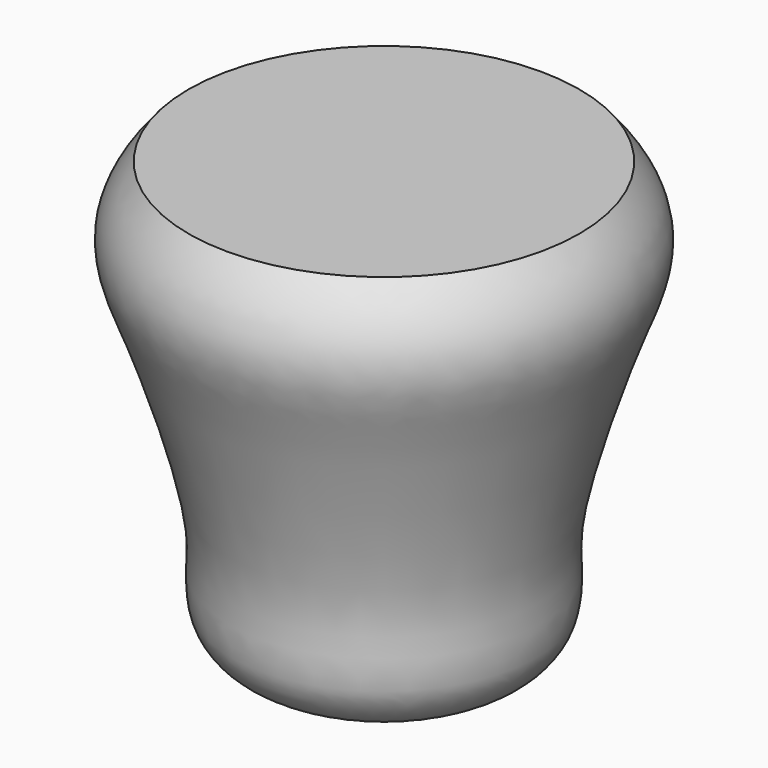
from build123d import *


with BuildPart() as f1:
    # F0 (on Right) → F1 (revolve)
    with BuildSketch(Plane.YZ):
        with BuildLine():
            Line((40, 90), (0, 90))
            Line((0, 90), (0, 0))
            Line((0, 0), (20, 0))
            add(Edge.make_bspline(
                [(40, 90), (49.5818336765, 78.8694407024), (42.4350350409, 64.2002089946), (33.3484499065, 35.488516994), (30.97101949, 21.463351906), (32.5174405975, 10.4827954865), (28.1788393461, 2.3869152735), (20, 0)],
                knots=[0, 0, 0, 0, 0.2424772002, 0.4945795444, 0.6684590037, 0.8145470688, 1, 1, 1, 1], degree=3))
        make_face()
    revolve(axis=Axis((0, 0, 45.4456442967), (0, 0, 1)))


solid = f1.part
